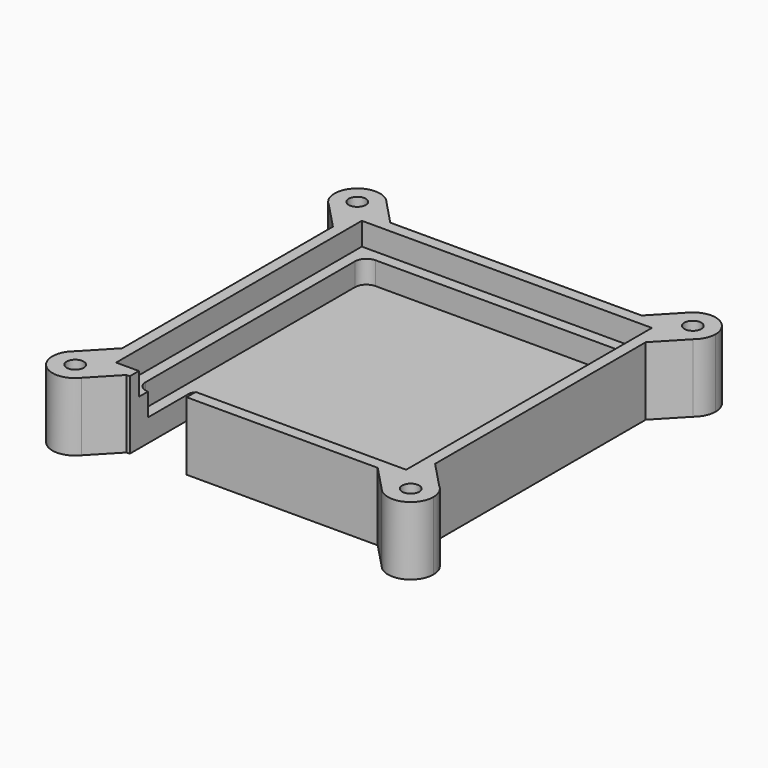
from build123d import *

# Parameters (mm, degrees)
F0_W      = 55
F0_H      = 58
F1_DEPTH  = 4
F2_W      = 55
F2_H      = 58
F2_W_2    = 47
F2_H_2    = 50
F3_DEPTH  = 8
F4_R      = 2
F5_W      = 10
F5_H      = 10
F6_DEPTH  = 25.4
F7_W      = 10
F7_H      = 4
F8_DEPTH  = 17.018
F9_R      = 1
F11_DEPTH = 4
F13_DEPTH = 12
F14_R     = 2.5
F15_DEPTH = 4
F16_R     = 1.5
F17_DEPTH = 25.4


# Not quite as in the source:
# - a feature names something its author has since deleted; it is built from what else it names


with BuildPart() as f1:
    # F0 (on Top) → F1 (new body)
    with BuildSketch(Plane.XY):
        Rectangle(F0_W, F0_H)
    extrude(amount=F1_DEPTH)

    # F2 (on face) → F3 (join)
    with BuildSketch(Plane.XY.offset(4)):
        Rectangle(F2_W, F2_H)
        Rectangle(F2_W_2, F2_H_2, mode=Mode.SUBTRACT)
    extrude(amount=F3_DEPTH)

    # F4
    f4_edges = [f1.edges().sort_by_distance(p)[0] for p in [
        (23.5, -25, 8),
        (-23.5, -25, 8),
        (-23.5, 25, 8),
        (23.5, 25, 8),
    ]]
    fillet(f4_edges, radius=F4_R)

    # F5 (on face) → F6 (cut)
    with BuildSketch(Plane.XY.offset(12)):
        with Locations((-16.5, -20)):
            Rectangle(F5_W, F5_H)
    extrude(amount=-F6_DEPTH, mode=Mode.SUBTRACT)

    # F7 (on face) → F8 (cut)
    with BuildSketch(Plane.XY.offset(12)):
        with Locations((-16.5, -27)):
            Rectangle(F7_W, F7_H)
    extrude(amount=-F8_DEPTH, mode=Mode.SUBTRACT)

    # F9
    f9_edges = [f1.edges().sort_by_distance(p)[0] for p in [
        (-21.5, -15, 2),
        (-11.5, -15, 2),
    ]]
    fillet(f9_edges, radius=F9_R)

    # F10 (on face) → F11 (cut)
    with BuildSketch(Plane.XY.offset(12)):
        with BuildLine():
            Line((25.5, -27), (25.5, 27))
            Line((25.5, 27), (-25.5, 27))
            Line((-25.5, 27), (-25.5, -27))
            Line((-25.5, -27), (-21.5, -27))
            Line((-21.5, -27), (-21.5, -25))
            ThreePointArc((-21.5, -25), (-22.9142135624, -24.4142135624), (-23.5, -23))
            Line((-23.5, -23), (-23.5, 23))
            ThreePointArc((-23.5, 23), (-22.9142135624, 24.4142135624), (-21.5, 25))
            Line((-21.5, 25), (21.5, 25))
            ThreePointArc((21.5, 25), (22.9142135624, 24.4142135624), (23.5, 23))
            Line((23.5, 23), (23.5, -23))
            ThreePointArc((23.5, -23), (22.9142135624, -24.4142135624), (21.5, -25))
            Line((21.5, -25), (-11.5, -25))
            Line((-11.5, -25), (-11.5, -27))
            Line((-11.5, -27), (25.5, -27))
        make_face()
    extrude(amount=-F11_DEPTH, mode=Mode.SUBTRACT)

    # F12 (on face) → F13 (join)
    with BuildSketch(Plane(origin=(0, 0, 0), x_dir=(1, 0, 0), z_dir=(0, 0, -1))):
        with BuildLine():
            ThreePointArc((-26.0358983849, 29), (-25.6362966948, 29.9647238196), (-25.5, 31))
            ThreePointArc((-25.5, 31), (-25.7257453718, 32.3247648854), (-26.3775010008, 33.5))
            Line((-26.3775010008, 33.5), (-32, 33.5))
            Line((-32, 33.5), (-32, 27.8775010008))
            ThreePointArc((-32, 27.8775010008), (-29.8027756377, 27.011475597), (-27.5, 27.5358983849))
            Line((-27.5, 27.5358983849), (-27.5, 29))
            Line((-27.5, 29), (-26.0358983849, 29))
        make_face()
        with BuildLine():
            Line((-32, 33.5), (-26.3775010008, 33.5))
            ThreePointArc((-26.3775010008, 33.5), (-32.3284271247, 33.8284271247), (-32, 27.8775010008))
            Line((-32, 27.8775010008), (-32, 33.5))
        make_face()
        with BuildLine():
            ThreePointArc((-27.5, 27.5358983849), (-29.8027756377, 27.011475597), (-32, 27.8775010008))
            Line((-32, 27.8775010008), (-27.5, 23.1462475253))
            Line((-27.5, 23.1462475253), (-27.5, 27.5358983849))
        make_face()
        with BuildLine():
            ThreePointArc((-26.3775010008, 33.5), (-25.7257453718, 32.3247648854), (-25.5, 31))
            ThreePointArc((-25.5, 31), (-25.6362966948, 29.9647238196), (-26.0358983849, 29))
            Line((-26.0358983849, 29), (-22.0974513047, 29))
            Line((-22.0974513047, 29), (-26.3775010008, 33.5))
        make_face()
        with BuildLine():
            Line((32, 33.5), (26.3775010008, 33.5))
            ThreePointArc((26.3775010008, 33.5), (25.511475597, 31.3027756377), (26.0358983849, 29))
            Line((26.0358983849, 29), (27.5, 29))
            Line((27.5, 29), (27.5, 27.5358983849))
            ThreePointArc((27.5, 27.5358983849), (29.8027756377, 27.011475597), (32, 27.8775010008))
            Line((32, 27.8775010008), (32, 33.5))
        make_face()
        with BuildLine():
            ThreePointArc((33.5, 31), (30.8247648854, 34.7742546282), (26.3775010008, 33.5))
            Line((26.3775010008, 33.5), (32, 33.5))
            Line((32, 33.5), (32, 27.8775010008))
            ThreePointArc((32, 27.8775010008), (33.1055512755, 29.2679491924), (33.5, 31))
        make_face()
        with BuildLine():
            Line((27.5, 23.1462475253), (32, 27.8775010008))
            ThreePointArc((32, 27.8775010008), (29.8027756377, 27.011475597), (27.5, 27.5358983849))
            Line((27.5, 27.5358983849), (27.5, 23.1462475253))
        make_face()
        with BuildLine():
            ThreePointArc((26.0358983849, 29), (25.511475597, 31.3027756377), (26.3775010008, 33.5))
            Line((26.3775010008, 33.5), (22.0974513047, 29))
            Line((22.0974513047, 29), (26.0358983849, 29))
        make_face()
        with BuildLine():
            ThreePointArc((-27.5, -27.5358983849), (-29.8027756377, -27.011475597), (-32, -27.8775010008))
            Line((-32, -27.8775010008), (-32, -33.5))
            Line((-32, -33.5), (-26.3775010008, -33.5))
            ThreePointArc((-26.3775010008, -33.5), (-25.7257453718, -32.3247648854), (-25.5, -31))
            ThreePointArc((-25.5, -31), (-25.6362966948, -29.9647238196), (-26.0358983849, -29))
            Line((-26.0358983849, -29), (-27.5, -29))
            Line((-27.5, -29), (-27.5, -27.5358983849))
        make_face()
        with BuildLine():
            Line((-32, -33.5), (-32, -27.8775010008))
            ThreePointArc((-32, -27.8775010008), (-32.3284271247, -33.8284271247), (-26.3775010008, -33.5))
            Line((-26.3775010008, -33.5), (-32, -33.5))
        make_face()
        with BuildLine():
            Line((-27.5, -23.1462475253), (-32, -27.8775010008))
            ThreePointArc((-32, -27.8775010008), (-29.8027756377, -27.011475597), (-27.5, -27.5358983849))
            Line((-27.5, -27.5358983849), (-27.5, -23.1462475253))
        make_face()
        with BuildLine():
            ThreePointArc((-25.5, -31), (-25.7257453718, -32.3247648854), (-26.3775010008, -33.5))
            Line((-26.3775010008, -33.5), (-22.0974513047, -29))
            Line((-22.0974513047, -29), (-26.0358983849, -29))
            ThreePointArc((-26.0358983849, -29), (-25.6362966948, -29.9647238196), (-25.5, -31))
        make_face()
        with BuildLine():
            ThreePointArc((26.0358983849, -29), (25.511475597, -31.3027756377), (26.3775010008, -33.5))
            Line((26.3775010008, -33.5), (32, -33.5))
            Line((32, -33.5), (32, -27.8775010008))
            ThreePointArc((32, -27.8775010008), (29.8027756377, -27.011475597), (27.5, -27.5358983849))
            Line((27.5, -27.5358983849), (27.5, -29))
            Line((27.5, -29), (26.0358983849, -29))
        make_face()
        with BuildLine():
            Line((22.0974513047, -29), (26.3775010008, -33.5))
            ThreePointArc((26.3775010008, -33.5), (25.511475597, -31.3027756377), (26.0358983849, -29))
            Line((26.0358983849, -29), (22.0974513047, -29))
        make_face()
        with BuildLine():
            ThreePointArc((27.5, -27.5358983849), (29.8027756377, -27.011475597), (32, -27.8775010008))
            Line((32, -27.8775010008), (27.5, -23.1462475253))
            Line((27.5, -23.1462475253), (27.5, -27.5358983849))
        make_face()
        with BuildLine():
            Line((32, -33.5), (26.3775010008, -33.5))
            ThreePointArc((26.3775010008, -33.5), (30.8247648854, -34.7742546282), (33.5, -31))
            ThreePointArc((33.5, -31), (33.1055512755, -29.2679491924), (32, -27.8775010008))
            Line((32, -27.8775010008), (32, -33.5))
        make_face()
    extrude(amount=-F13_DEPTH)

    # F14 (on face) → F15 (cut)
    with BuildSketch(Plane(origin=(0, 0, 0), x_dir=(1, 0, 0), z_dir=(0, 0, -1))):
        with Locations((-29.5, -31)):
            Circle(F14_R)
        with Locations((29.5, -31)):
            Circle(F14_R)
        with Locations((-29.5, 31)):
            Circle(F14_R)
        with Locations((29.5, 31)):
            Circle(F14_R)
    extrude(amount=-F15_DEPTH, mode=Mode.SUBTRACT)

    # F16 (on face) → F17 (cut)
    with BuildSketch(Plane.XY.offset(12)):
        with Locations((29.5, -31)):
            Circle(F16_R)
        with Locations((-29.5, -31)):
            Circle(F16_R)
        with Locations((29.5, 31)):
            Circle(F16_R)
        with Locations((-29.5, 31)):
            Circle(F16_R)
    extrude(amount=-F17_DEPTH, mode=Mode.SUBTRACT)


solid = f1.part
